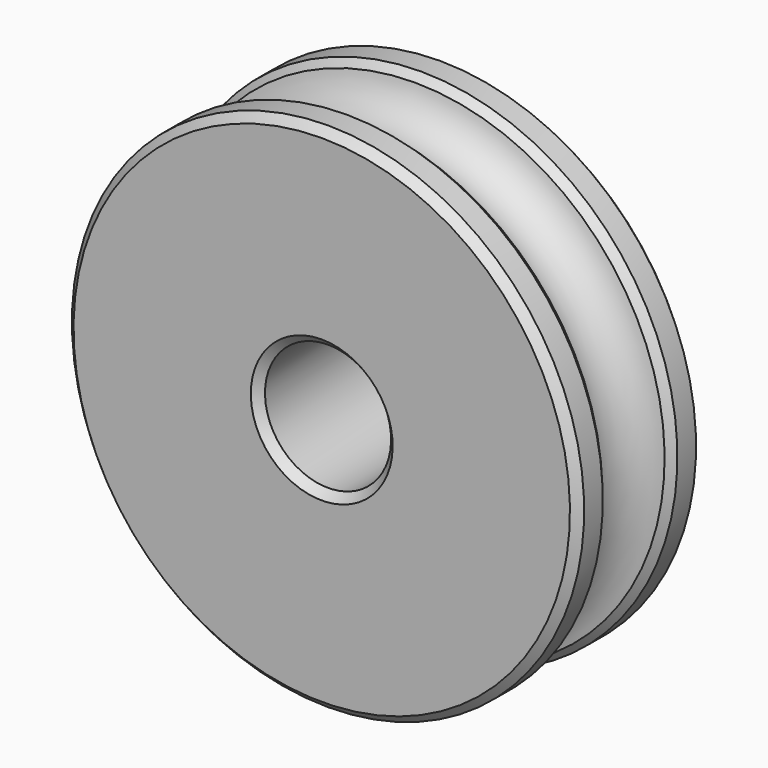
from build123d import *


# Not quite as in the source:
# - a fillet or chamfer that OpenCascade refuses, or shapes differently, is made with other operations: its cross-section is extruded or revolved along the edge and cut away or added


with BuildPart() as f1:
    # F0 (on Right) → F1 (revolve)
    with BuildSketch(Plane.YZ):
        with BuildLine():
            Line((-1.975, 1.6), (0, 1.6))
            Line((0, 1.6), (1.975, 1.6))
            Line((1.975, 1.6), (1.975, 6.5))
            Line((1.975, 6.5), (1, 6.5))
            ThreePointArc((1, 6.5), (0, 5.5), (-1, 6.5))
            Line((-1, 6.5), (-1.975, 6.5))
            Line((-1.975, 6.5), (-1.975, 1.6))
        make_face()
    revolve(axis=Axis((0, 2.5333669037, 0), (0, 1, 0)))

    # F2: chamfer of 0.2 on 9 edges, made by hand

    # F2_s1 → F2_t2 (revolve, cut)
    with BuildSketch(Plane.YZ):
        Polygon((-1.775, 1.6), (-1.975, 1.8), (-1.975, 1.6), align=None)
    revolve(axis=Axis((0, -1.975, 0), (0, 1, 0)), mode=Mode.SUBTRACT)

    # F2_s3 → F2_t4 (revolve, cut)
    with BuildSketch(Plane.YZ):
        Polygon((1.775, 1.6), (1.975, 1.8), (1.975, 1.6), align=None)
    revolve(axis=Axis((0, 1.975, 0), (0, 1, 0)), mode=Mode.SUBTRACT)

    # F2_s5 → F2_t6 (revolve, cut)
    with BuildSketch(Plane.YZ):
        with BuildLine():
            Line((-0.9860132972, 6.3333333333), (-1.1832159566, 6.5))
            Line((-1.1832159566, 6.5), (-1, 6.5))
            ThreePointArc((-1, 6.5), (-0.9962551156, 6.4135376119), (-0.9860132972, 6.3333333333))
        make_face()
    revolve(axis=Axis((0, -1, 0), (0, 1, 0)), mode=Mode.SUBTRACT)

    # F2_s7 → F2_t8 (revolve, cut)
    with BuildSketch(Plane.YZ):
        Polygon((-1.775, 6.5), (-1.975, 6.3), (-1.975, 6.5), align=None)
    revolve(axis=Axis((0, -1.975, 0), (0, 1, 0)), mode=Mode.SUBTRACT)

    # F2_s9 → F2_t10 (revolve, cut)
    with BuildSketch(Plane.YZ):
        Polygon((1.975, 6.3), (1.775, 6.5), (1.975, 6.5), align=None)
    revolve(axis=Axis((0, 1.975, 0), (0, 1, 0)), mode=Mode.SUBTRACT)

    # F2_s11 → F2_t12 (revolve, cut)
    with BuildSketch(Plane.YZ):
        with BuildLine():
            Line((1.1832159566, 6.5), (0.9860132972, 6.3333333333))
            ThreePointArc((0.9860132972, 6.3333333333), (0.9962551156, 6.4135376119), (1, 6.5))
            Line((1, 6.5), (1.1832159566, 6.5))
        make_face()
    revolve(axis=Axis((0, 1, 0), (0, 1, 0)), mode=Mode.SUBTRACT)


solid = f1.part
